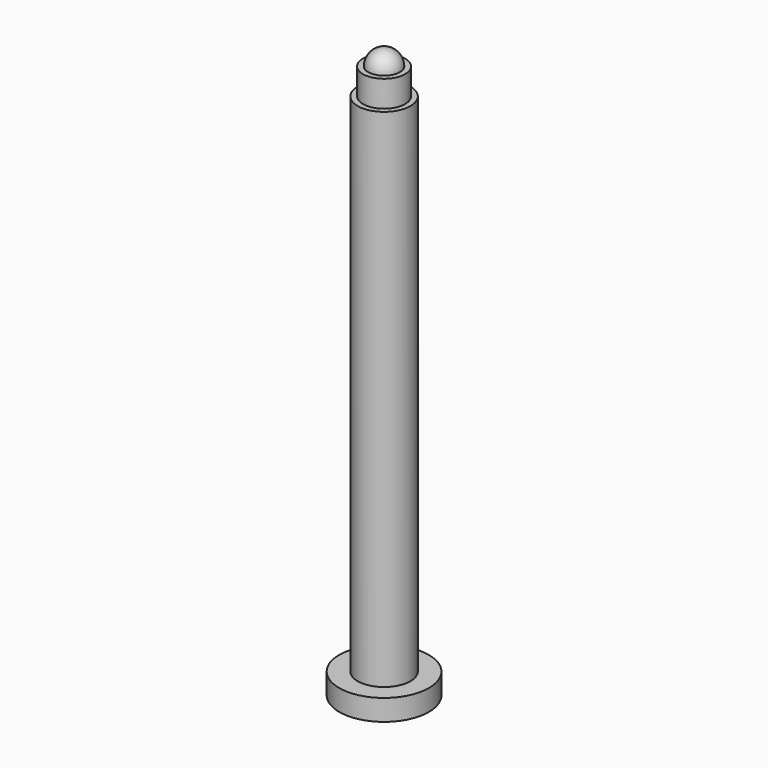
from build123d import *

# Parameters (mm, degrees)
F0_R         = 8.5
F1_DEPTH     = 4
F2_R         = 5
F3_DEPTH     = 100
F4_W         = 4
F4_H         = 5
F8_TEXT_SIZE = 9.1589025109
F9_DEPTH     = 0.1


# Not quite as in the source:
# - Text() gives the source's letters only with a copy of the font that has no kerning and outlines rounded to 1/6400 em; it was checked with that copy


with BuildPart() as f1:
    # F0 (on Top) → F1 (new body)
    with BuildSketch(Plane.XY):
        Circle(F0_R)
    extrude(amount=F1_DEPTH)

    # F2 (on Top) → F3 (join)
    with BuildSketch(Plane.XY):
        Circle(F2_R)
    extrude(amount=F3_DEPTH)

    # F4 (on Right) → F5 (revolve)
    with BuildSketch(Plane.YZ):
        with Locations((2, 102.5)):
            Rectangle(F4_W, F4_H)
    revolve(axis=Axis((0, 0, 102.5), (0, 0, -1)))

    # F6 (on Right) → F7 (revolve)
    with BuildSketch(Plane.YZ):
        with BuildLine():
            ThreePointArc((3, 105), (2.1213203436, 107.1213203436), (0, 108))
            Line((0, 108), (0, 105))
            Line((0, 105), (3, 105))
        make_face()
    revolve(axis=Axis((0, 0, 106.5), (0, 0, -1)))

    # F8 (on face) → F9 (cut)
    with BuildSketch(Plane(origin=(0, 0, 0), x_dir=(1, 0, 0), z_dir=(0, 0, -1))):
        with Locations((-7.8344393431, -3.2972049039)):
            Text('E02', F8_TEXT_SIZE, font='Open Sans', text_align=(TextAlign.LEFT, TextAlign.BOTTOM))
    extrude(amount=-F9_DEPTH, mode=Mode.SUBTRACT)


solid = f1.part
